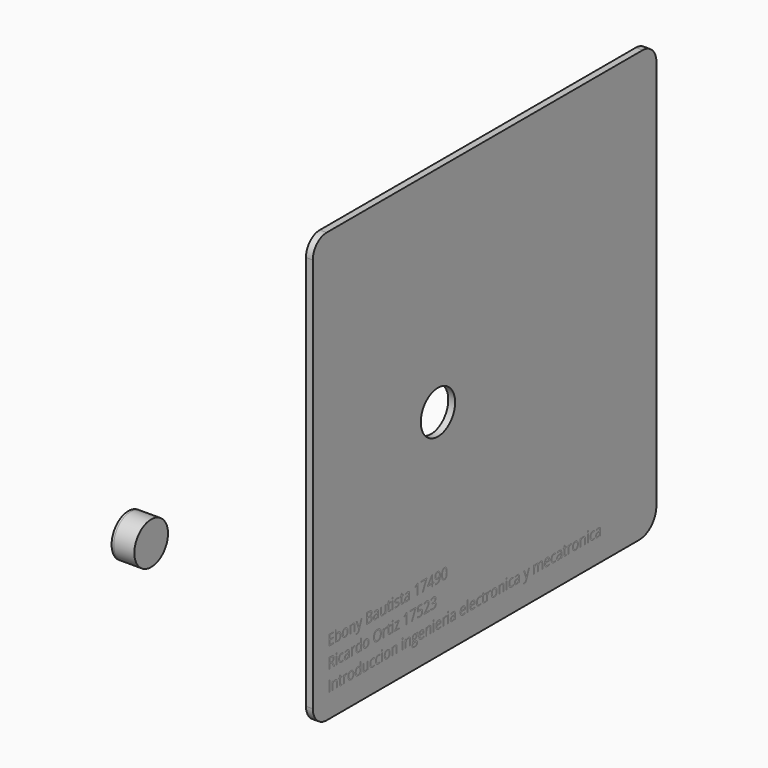
from build123d import *

# Parameters (mm, degrees)
F0_W         = 200
F0_H         = 200
F0_R         = 10
F1_DEPTH     = 3.2
F2_R         = 8
F3_R         = 9.8
F4_DEPTH     = 9.6
F5_R         = 10
F3_TEXT_SIZE = 6.9444444444
F6_DEPTH     = 1


# Not quite as in the source:
# - Text() gives the source's letters only with a copy of the font that has no kerning and outlines rounded to 1/6400 em; it was checked with that copy


with BuildPart() as f1:
    # F0 (on Right) → F1 (new body)
    with BuildSketch(Plane.YZ):
        with Locations((-18, 0)):
            Rectangle(F0_W, F0_H)
        with Locations((-45.17, 0)):
            Circle(F0_R, mode=Mode.SUBTRACT)
    extrude(amount=F1_DEPTH)

    # F2
    f2_edges = [f1.edges().sort_by_distance(p)[0] for p in [
        (1.6, -118, 100),
        (1.6, -118, -100),
        (1.6, 82, 100),
    ]]
    fillet(f2_edges, radius=F2_R)

    # F5
    f5_edges = [f1.edges().sort_by_distance(p)[0] for p in [
        (1.6, 82, -100),
    ]]
    fillet(f5_edges, radius=F5_R)


with BuildPart() as f4:
    # F3 (on face) → F4 (new body)
    with BuildSketch(Plane.YZ.offset(3.2)):
        with Locations((-224.1166979074, 22.1441891044)):
            Circle(F3_R)
    extrude(amount=F4_DEPTH)


with BuildPart() as f6:
    # F3 (on face) → F6 (new body)
    with BuildSketch(Plane.YZ.offset(3.2)):
        with Locations((-224.1166979074, 22.1441891044)):
            Circle(F3_R)
        with Locations((-109.3953326344, -70.2321949601)):
            Text('Ebony Bautista 17490', F3_TEXT_SIZE, font='Open Sans', text_align=(TextAlign.LEFT, TextAlign.BOTTOM))
        with Locations((-109.3953326344, -79.6766394046)):
            Text('Ricardo Ortiz 17523', F3_TEXT_SIZE, font='Open Sans', text_align=(TextAlign.LEFT, TextAlign.BOTTOM))
        with Locations((-109.3953326344, -89.121083849)):
            Text('Introduccion ingenieria electronica y mecatronica', F3_TEXT_SIZE, font='Open Sans', text_align=(TextAlign.LEFT, TextAlign.BOTTOM))
    extrude(amount=-F6_DEPTH)


solid = Compound([f1.part, f4.part, f6.part])
